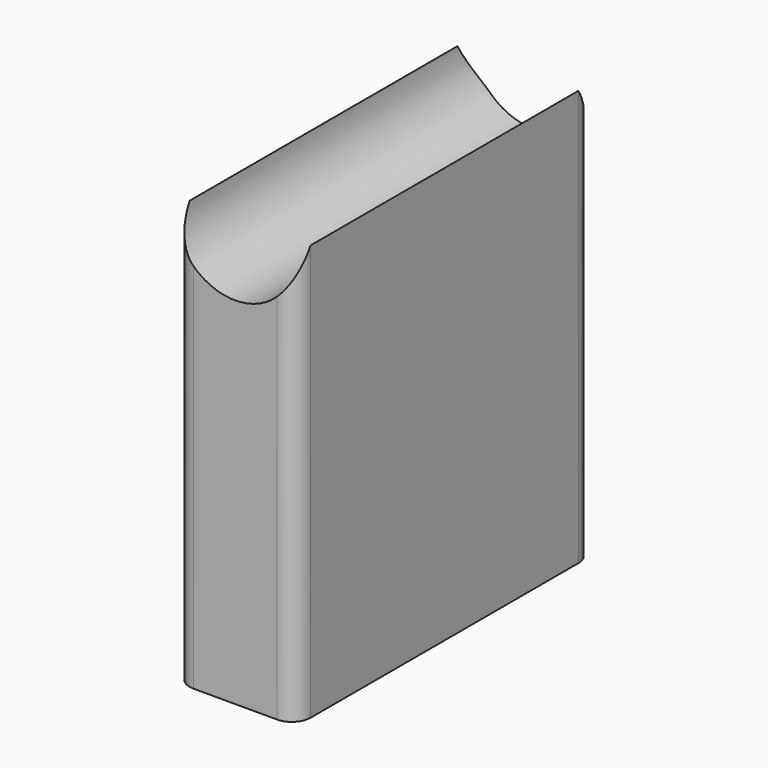
from build123d import *

# Parameters (mm, degrees)
F0_W        = 6.5
F0_H        = 20
F1_DEPTH    = 22.35
F3_DEPTH    = 25
F4_T1_DEPTH = 27.35


# Not quite as in the source:
# - a fillet or chamfer that OpenCascade refuses, or shapes differently, is made with other operations: its cross-section is extruded or revolved along the edge and cut away or added


with BuildPart() as f1:
    # F0 (on Top) → F1 (new body)
    with BuildSketch(Plane.XY):
        with Locations((3.25, 10)):
            Rectangle(F0_W, F0_H)
    extrude(amount=F1_DEPTH)

    # F2 (on face) → F3 (cut)
    with BuildSketch(Plane.XZ):
        with BuildLine():
            ThreePointArc((6.5, 22.35), (3.25, 25.6), (0, 22.35))
            Line((0, 22.35), (6.5, 22.35))
        make_face()
        with BuildLine():
            Line((6.5, 22.35), (0, 22.35))
            ThreePointArc((0, 22.35), (3.25, 19.1), (6.5, 22.35))
        make_face()
    extrude(amount=-F3_DEPTH, mode=Mode.SUBTRACT)

    # F4: fillet of radius 1 on 4 edges, made by hand

    # F4_s2 → F4_t1 (cut)
    with BuildSketch(Plane.XY.offset(-2.5)):
        with BuildLine():
            ThreePointArc((5.5, 0), (6.2071067812, 0.2928932188), (6.5, 1))
            Line((6.5, 1), (6.5, 0))
            Line((6.5, 0), (5.5, 0))
        make_face()
        with BuildLine():
            ThreePointArc((0, 1), (0.2928932188, 0.2928932188), (1, 0))
            Line((1, 0), (0, 0))
            Line((0, 0), (0, 1))
        make_face()
        with BuildLine():
            ThreePointArc((5.5, 20), (6.2071067812, 19.7071067812), (6.5, 19))
            Line((6.5, 19), (6.5, 20))
            Line((6.5, 20), (5.5, 20))
        make_face()
        with BuildLine():
            ThreePointArc((0, 19), (0.2928932188, 19.7071067812), (1, 20))
            Line((1, 20), (0, 20))
            Line((0, 20), (0, 19))
        make_face()
    extrude(amount=F4_T1_DEPTH, mode=Mode.SUBTRACT)


solid = f1.part
